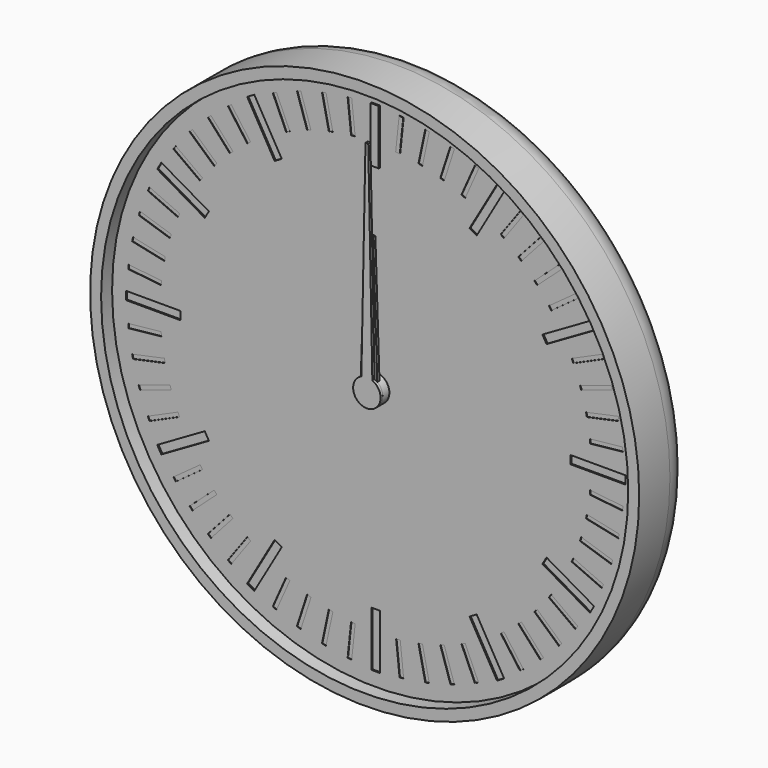
from build123d import *

# Parameters (mm, degrees)
F0_R      = 100
F1_DEPTH  = 24
F2_R      = 10
F3_T      = -4
F4_R      = 5
F4_R_2    = 3
F5_DEPTH  = 2
F6_DEPTH  = 19
F7_DEPTH  = 8
F9_DEPTH  = 4
F11_DEPTH = 4
F12_R     = 5
F12_R_2   = 3
F13_DEPTH = 2
F14_R     = 3
F15_DEPTH = 4
F17_DEPTH = 4
F18_R     = 3
F19_DEPTH = 2
F20_R     = 98
F20_R_2   = 5
F21_DEPTH = 1
F23_R     = 5
F23_R_2   = 3
F24_DEPTH = 2
F25_W     = 3
F25_H     = 20
F25_W_2   = 20
F25_H_2   = 3
F26_DEPTH = 0.5
F27_W     = 1.5
F27_H     = 12
F27_W_2   = 12
F27_H_2   = 1.5
F28_DEPTH = 0.2
F29_DEPTH = 1
F30_DEPTH = 0.4
F31_R     = 5
F31_R_2   = 3
F32_DEPTH = 5
F33_R     = 3
F34_DEPTH = 1
F36_DEPTH = 1


with BuildPart() as f1:
    # F0 (on Front) → F1 (new body)
    with BuildSketch(Plane.XZ):
        Circle(F0_R)
    extrude(amount=F1_DEPTH)

    # F2
    f2_edges = [f1.edges().sort_by_distance(p)[0] for p in [
        (-100, 0, 0),
    ]]
    fillet(f2_edges, radius=F2_R)

    # F3
    f3_openings = [f1.faces().sort_by_distance(p)[0] for p in [
        (0, -24, 0),
    ]]
    offset(amount=F3_T, openings=f3_openings)

    # F4 (on face) → F5 (join)
    with BuildSketch(Plane.XZ.offset(4)):
        Circle(F4_R)
        Circle(F4_R_2, mode=Mode.SUBTRACT)
        with Locations((40, 0)):
            Circle(F4_R)
        with Locations((40, 0)):
            Circle(F4_R_2, mode=Mode.SUBTRACT)
    extrude(amount=F5_DEPTH)


with BuildPart() as f6:
    # F6 (new): a face of the model
    f6_faces = [f1.part.faces().sort_by_distance(p)[0] for p in [
        (0, -4, 0),
    ]]
    extrude(f6_faces, amount=F6_DEPTH)

    # F8 (on face) → F9 (join)
    with BuildSketch(Plane.XZ.offset(6)):
        with BuildLine():
            ThreePointArc((9.2729637667, -1.3794085621), (9.3494561423, -0.6915886375), (9.375, 0))
            ThreePointArc((9.375, 0), (9.3494561423, 0.6915886375), (9.2729637667, 1.3794085621))
            ThreePointArc((9.2729637667, 1.3794085621), (8.9161548403, 2.8970343223), (8.3127812852, 4.3345463782))
            ThreePointArc((8.3127812852, 4.3345463782), (7.5845343223, 5.5104867402), (6.6911892658, 6.566476316))
            ThreePointArc((6.6911892658, 6.566476316), (5.5104867402, 7.5845343223), (4.1773988938, 8.3928519278))
            ThreePointArc((4.1773988938, 8.3928519278), (2.8970343223, 8.9161548403), (1.5536078905, 9.2453733036))
            ThreePointArc((1.5536078905, 9.2453733036), (0, 9.375), (-1.5536078905, 9.2453733036))
            ThreePointArc((-1.5536078905, 9.2453733036), (-2.8970343223, 8.9161548403), (-4.1773988938, 8.3928519278))
            ThreePointArc((-4.1773988938, 8.3928519278), (-5.5104867402, 7.5845343223), (-6.6911892658, 6.566476316))
            ThreePointArc((-6.6911892658, 6.566476316), (-7.5845343223, 5.5104867402), (-8.3127812852, 4.3345463782))
            ThreePointArc((-8.3127812852, 4.3345463782), (-8.9161548403, 2.8970343223), (-9.2729637667, 1.3794085621))
            ThreePointArc((-9.2729637667, 1.3794085621), (-9.375, 0), (-9.2729637667, -1.3794085621))
            ThreePointArc((-9.2729637667, -1.3794085621), (-8.9161548403, -2.8970343223), (-8.3127812852, -4.3345463782))
            ThreePointArc((-8.3127812852, -4.3345463782), (-7.5845343223, -5.5104867402), (-6.6911892658, -6.566476316))
            ThreePointArc((-6.6911892658, -6.566476316), (-5.5104867402, -7.5845343223), (-4.1773988938, -8.3928519278))
            ThreePointArc((-4.1773988938, -8.3928519278), (-2.8970343223, -8.9161548403), (-1.5536078905, -9.2453733036))
            ThreePointArc((-1.5536078905, -9.2453733036), (0, -9.375), (1.5536078905, -9.2453733036))
            ThreePointArc((1.5536078905, -9.2453733036), (2.8970343223, -8.9161548403), (4.1773988938, -8.3928519278))
            ThreePointArc((4.1773988938, -8.3928519278), (5.5104867402, -7.5845343223), (6.6911892658, -6.566476316))
            ThreePointArc((6.6911892658, -6.566476316), (7.5845343223, -5.5104867402), (8.3127812852, -4.3345463782))
            ThreePointArc((8.3127812852, -4.3345463782), (8.9161548403, -2.8970343223), (9.2729637667, -1.3794085621))
        make_face()
        with BuildLine():
            ThreePointArc((8.3127812852, 4.3345463782), (8.9161548403, 2.8970343223), (9.2729637667, 1.3794085621))
            Line((9.2729637667, 1.3794085621), (11.1823199426, 2.3946312492))
            Line((11.1823199426, 2.3946312492), (10.8182678729, 3.515068311))
            Line((10.8182678729, 3.515068311), (10.4542158031, 4.6355053728))
            Line((10.4542158031, 4.6355053728), (8.3127812852, 4.3345463782))
        make_face()
        with BuildLine():
            Line((11.1823199426, -2.3946312492), (9.2729637667, -1.3794085621))
            ThreePointArc((9.2729637667, -1.3794085621), (8.9161548403, -2.8970343223), (8.3127812852, -4.3345463782))
            Line((8.3127812852, -4.3345463782), (10.4542158031, -4.6355053728))
            Line((10.4542158031, -4.6355053728), (10.8182678729, -3.515068311))
            Line((10.8182678729, -3.515068311), (11.1823199426, -2.3946312492))
        make_face()
        with BuildLine():
            ThreePointArc((4.1773988938, 8.3928519278), (5.5104867402, 7.5845343223), (6.6911892658, 6.566476316))
            Line((6.6911892658, 6.566476316), (7.6391579371, 8.5101001246))
            Line((7.6391579371, 8.5101001246), (6.6860572448, 9.202568311))
            Line((6.6860572448, 9.202568311), (5.7329565525, 9.8950364974))
            Line((5.7329565525, 9.8950364974), (4.1773988938, 8.3928519278))
        make_face()
        with BuildLine():
            Line((7.6391579371, -8.5101001246), (6.6911892658, -6.566476316))
            ThreePointArc((6.6911892658, -6.566476316), (5.5104867402, -7.5845343223), (4.1773988938, -8.3928519278))
            Line((4.1773988938, -8.3928519278), (5.7329565525, -9.8950364974))
            Line((5.7329565525, -9.8950364974), (6.6860572448, -9.202568311))
            Line((6.6860572448, -9.202568311), (7.6391579371, -8.5101001246))
        make_face()
        with BuildLine():
            ThreePointArc((-1.5536078905, 9.2453733036), (0, 9.375), (1.5536078905, 9.2453733036))
            Line((1.5536078905, 9.2453733036), (1.1780972451, 11.375))
            Line((1.1780972451, 11.375), (0, 11.375))
            Line((0, 11.375), (-1.1780972451, 11.375))
            Line((-1.1780972451, 11.375), (-1.5536078905, 9.2453733036))
        make_face()
        with BuildLine():
            Line((1.1780972451, -11.375), (1.5536078905, -9.2453733036))
            ThreePointArc((1.5536078905, -9.2453733036), (0, -9.375), (-1.5536078905, -9.2453733036))
            Line((-1.5536078905, -9.2453733036), (-1.1780972451, -11.375))
            Line((-1.1780972451, -11.375), (0, -11.375))
            Line((0, -11.375), (1.1780972451, -11.375))
        make_face()
        with BuildLine():
            ThreePointArc((-6.6911892658, 6.566476316), (-5.5104867402, 7.5845343223), (-4.1773988938, 8.3928519278))
            Line((-4.1773988938, 8.3928519278), (-5.7329565525, 9.8950364974))
            Line((-5.7329565525, 9.8950364974), (-6.6860572448, 9.202568311))
            Line((-6.6860572448, 9.202568311), (-7.6391579371, 8.5101001246))
            Line((-7.6391579371, 8.5101001246), (-6.6911892658, 6.566476316))
        make_face()
        with BuildLine():
            Line((-5.7329565525, -9.8950364974), (-4.1773988938, -8.3928519278))
            ThreePointArc((-4.1773988938, -8.3928519278), (-5.5104867402, -7.5845343223), (-6.6911892658, -6.566476316))
            Line((-6.6911892658, -6.566476316), (-7.6391579371, -8.5101001246))
            Line((-7.6391579371, -8.5101001246), (-6.6860572448, -9.202568311))
            Line((-6.6860572448, -9.202568311), (-5.7329565525, -9.8950364974))
        make_face()
        with BuildLine():
            ThreePointArc((-9.2729637667, 1.3794085621), (-8.9161548403, 2.8970343223), (-8.3127812852, 4.3345463782))
            Line((-8.3127812852, 4.3345463782), (-10.4542158031, 4.6355053728))
            Line((-10.4542158031, 4.6355053728), (-10.8182678729, 3.515068311))
            Line((-10.8182678729, 3.515068311), (-11.1823199426, 2.3946312492))
            Line((-11.1823199426, 2.3946312492), (-9.2729637667, 1.3794085621))
        make_face()
        with BuildLine():
            Line((-10.4542158031, -4.6355053728), (-8.3127812852, -4.3345463782))
            ThreePointArc((-8.3127812852, -4.3345463782), (-8.9161548403, -2.8970343223), (-9.2729637667, -1.3794085621))
            Line((-9.2729637667, -1.3794085621), (-11.1823199426, -2.3946312492))
            Line((-11.1823199426, -2.3946312492), (-10.8182678729, -3.515068311))
            Line((-10.8182678729, -3.515068311), (-10.4542158031, -4.6355053728))
        make_face()
    extrude(amount=F9_DEPTH)

    # F35 (on face) → F36 (join)
    with BuildSketch(Plane.XZ.offset(23)):
        with BuildLine():
            ThreePointArc((-2, 4.582575695), (-2.7386127875, -4.1833001327), (5, 0))
            ThreePointArc((5, 0), (4.1833001327, 2.7386127875), (2, 4.582575695))
            ThreePointArc((2, 4.582575695), (0, 5), (-2, 4.582575695))
        make_face()
        with BuildLine():
            ThreePointArc((-2, 4.582575695), (0, 5), (2, 4.582575695))
            Line((2, 4.582575695), (0.5, 80))
            Line((0.5, 80), (0, 80))
            Line((0, 80), (-0.5, 80))
            Line((-0.5, 80), (-2, 4.582575695))
        make_face()
    extrude(amount=-F36_DEPTH)


with BuildPart() as f7:
    # F7 (new): a face of the model
    f7_faces = [f1.part.faces().sort_by_distance(p)[0] for p in [
        (40, -4, 0),
    ]]
    extrude(f7_faces, amount=F7_DEPTH)

    # F10 (on face) → F11 (join)
    with BuildSketch(Plane.XZ.offset(6)):
        with BuildLine():
            ThreePointArc((68.0829066802, -1.5381733945), (68.1144747006, -0.7693746225), (68.125, 0))
            ThreePointArc((68.125, 0), (68.1144747006, 0.7693746225), (68.0829066802, 1.5381733945))
            ThreePointArc((68.0829066802, 1.5381733945), (67.9709283072, 2.9398630294), (67.7890320221, 4.3342039956))
            ThreePointArc((67.7890320221, 4.3342039956), (67.5104012706, 5.8475163042), (67.1494235596, 7.3433252263))
            ThreePointArc((67.1494235596, 7.3433252263), (66.7484645208, 8.6911029668), (66.280643318, 10.0171558733))
            ThreePointArc((66.280643318, 10.0171558733), (65.6934659962, 11.4394680865), (65.0293803521, 12.8275385085))
            ThreePointArc((65.0293803521, 12.8275385085), (64.3569644814, 14.0625), (63.6236643925, 15.2623099717))
            ThreePointArc((63.6236643925, 15.2623099717), (62.7536029668, 16.5314602207), (61.815433119, 17.7511268046))
            ThreePointArc((61.815433119, 17.7511268046), (60.9009482166, 18.8192983038), (59.934217974, 19.8404278876))
            ThreePointArc((59.934217974, 19.8404278876), (58.8192983038, 20.9009482166), (57.6480467764, 21.8989056799))
            ThreePointArc((57.6480467764, 21.8989056799), (56.5314602207, 22.7536029668), (55.3735505752, 23.5514238999))
            ThreePointArc((55.3735505752, 23.5514238999), (54.0625, 24.3569644814), (52.709356105, 25.0895972944))
            ThreePointArc((52.709356105, 25.0895972944), (51.4394680865, 25.6934659962), (50.1409852457, 26.2331096755))
            ThreePointArc((50.1409852457, 26.2331096755), (48.6911029668, 26.7484645208), (47.2152055856, 27.1837531139))
            ThreePointArc((47.2152055856, 27.1837531139), (45.8475163042, 27.5104012706), (44.4652101991, 27.7682826779))
            ThreePointArc((44.4652101991, 27.7682826779), (42.9398630294, 27.9709283072), (41.4057159597, 28.0898484802))
            ThreePointArc((41.4057159597, 28.0898484802), (40, 28.125), (38.5942840403, 28.0898484802))
            ThreePointArc((38.5942840403, 28.0898484802), (37.0601369706, 27.9709283072), (35.5347898009, 27.7682826779))
            ThreePointArc((35.5347898009, 27.7682826779), (34.1524836958, 27.5104012706), (32.7847944144, 27.1837531139))
            ThreePointArc((32.7847944144, 27.1837531139), (31.3088970332, 26.7484645208), (29.8590147543, 26.2331096755))
            ThreePointArc((29.8590147543, 26.2331096755), (28.5605319135, 25.6934659962), (27.290643895, 25.0895972944))
            ThreePointArc((27.290643895, 25.0895972944), (25.9375, 24.3569644814), (24.6264494248, 23.5514238999))
            ThreePointArc((24.6264494248, 23.5514238999), (23.4685397793, 22.7536029668), (22.3519532236, 21.8989056799))
            ThreePointArc((22.3519532236, 21.8989056799), (21.1807016962, 20.9009482166), (20.065782026, 19.8404278876))
            ThreePointArc((20.065782026, 19.8404278876), (19.0990517834, 18.8192983038), (18.184566881, 17.7511268046))
            ThreePointArc((18.184566881, 17.7511268046), (17.2463970332, 16.5314602207), (16.3763356075, 15.2623099717))
            ThreePointArc((16.3763356075, 15.2623099717), (15.6430355186, 14.0625), (14.9706196479, 12.8275385085))
            ThreePointArc((14.9706196479, 12.8275385085), (14.3065340038, 11.4394680865), (13.719356682, 10.0171558733))
            ThreePointArc((13.719356682, 10.0171558733), (13.2515354792, 8.6911029668), (12.8505764404, 7.3433252263))
            ThreePointArc((12.8505764404, 7.3433252263), (12.4895987294, 5.8475163042), (12.2109679779, 4.3342039956))
            ThreePointArc((12.2109679779, 4.3342039956), (12.0290716928, 2.9398630294), (11.9170933198, 1.5381733945))
            ThreePointArc((11.9170933198, 1.5381733945), (11.875, 0), (11.9170933198, -1.5381733945))
            ThreePointArc((11.9170933198, -1.5381733945), (12.0290716928, -2.9398630294), (12.2109679779, -4.3342039956))
            ThreePointArc((12.2109679779, -4.3342039956), (12.4895987294, -5.8475163042), (12.8505764404, -7.3433252263))
            ThreePointArc((12.8505764404, -7.3433252263), (13.2515354792, -8.6911029668), (13.719356682, -10.0171558733))
            ThreePointArc((13.719356682, -10.0171558733), (14.3065340038, -11.4394680865), (14.9706196479, -12.8275385085))
            ThreePointArc((14.9706196479, -12.8275385085), (15.6430355186, -14.0625), (16.3763356075, -15.2623099717))
            ThreePointArc((16.3763356075, -15.2623099717), (17.2463970332, -16.5314602207), (18.184566881, -17.7511268046))
            ThreePointArc((18.184566881, -17.7511268046), (19.0990517834, -18.8192983038), (20.065782026, -19.8404278876))
            ThreePointArc((20.065782026, -19.8404278876), (21.1807016962, -20.9009482166), (22.3519532236, -21.8989056799))
            ThreePointArc((22.3519532236, -21.8989056799), (23.4685397793, -22.7536029668), (24.6264494248, -23.5514238999))
            ThreePointArc((24.6264494248, -23.5514238999), (25.9375, -24.3569644814), (27.290643895, -25.0895972944))
            ThreePointArc((27.290643895, -25.0895972944), (28.5605319135, -25.6934659962), (29.8590147543, -26.2331096755))
            ThreePointArc((29.8590147543, -26.2331096755), (31.3088970332, -26.7484645208), (32.7847944144, -27.1837531139))
            ThreePointArc((32.7847944144, -27.1837531139), (34.1524836958, -27.5104012706), (35.5347898009, -27.7682826779))
            ThreePointArc((35.5347898009, -27.7682826779), (37.0601369706, -27.9709283072), (38.5942840403, -28.0898484802))
            ThreePointArc((38.5942840403, -28.0898484802), (40, -28.125), (41.4057159597, -28.0898484802))
            ThreePointArc((41.4057159597, -28.0898484802), (42.9398630294, -27.9709283072), (44.4652101991, -27.7682826779))
            ThreePointArc((44.4652101991, -27.7682826779), (45.8475163042, -27.5104012706), (47.2152055856, -27.1837531139))
            ThreePointArc((47.2152055856, -27.1837531139), (48.6911029668, -26.7484645208), (50.1409852457, -26.2331096755))
            ThreePointArc((50.1409852457, -26.2331096755), (51.4394680865, -25.6934659962), (52.709356105, -25.0895972944))
            ThreePointArc((52.709356105, -25.0895972944), (54.0625, -24.3569644814), (55.3735505752, -23.5514238999))
            ThreePointArc((55.3735505752, -23.5514238999), (56.5314602207, -22.7536029668), (57.6480467764, -21.8989056799))
            ThreePointArc((57.6480467764, -21.8989056799), (58.8192983038, -20.9009482166), (59.934217974, -19.8404278876))
            ThreePointArc((59.934217974, -19.8404278876), (60.9009482166, -18.8192983038), (61.815433119, -17.7511268046))
            ThreePointArc((61.815433119, -17.7511268046), (62.7536029668, -16.5314602207), (63.6236643925, -15.2623099717))
            ThreePointArc((63.6236643925, -15.2623099717), (64.3569644814, -14.0625), (65.0293803521, -12.8275385085))
            ThreePointArc((65.0293803521, -12.8275385085), (65.6934659962, -11.4394680865), (66.280643318, -10.0171558733))
            ThreePointArc((66.280643318, -10.0171558733), (66.7484645208, -8.6911029668), (67.1494235596, -7.3433252263))
            ThreePointArc((67.1494235596, -7.3433252263), (67.5104012706, -5.8475163042), (67.7890320221, -4.3342039956))
            ThreePointArc((67.7890320221, -4.3342039956), (67.9709283072, -2.9398630294), (68.0829066802, -1.5381733945))
        make_face()
        with BuildLine():
            ThreePointArc((68.0829066802, 1.5381733945), (68.1144747006, 0.7693746225), (68.125, 0))
            ThreePointArc((68.125, 0), (68.1144747006, -0.7693746225), (68.0829066802, -1.5381733945))
            Line((68.0829066802, -1.5381733945), (70.125, -1.1780972451))
            Line((70.125, -1.1780972451), (70.125, 0))
            Line((70.125, 0), (70.125, 1.1780972451))
            Line((70.125, 1.1780972451), (68.0829066802, 1.5381733945))
        make_face()
        with BuildLine():
            ThreePointArc((67.1494235596, 7.3433252263), (67.5104012706, 5.8475163042), (67.7890320221, 4.3342039956))
            Line((67.7890320221, 4.3342039956), (69.7116366623, 5.1109866922))
            Line((69.7116366623, 5.1109866922), (69.4666964721, 6.2633396859))
            Line((69.4666964721, 6.2633396859), (69.2217562819, 7.4156926796))
            Line((69.2217562819, 7.4156926796), (67.1494235596, 7.3433252263))
        make_face()
        with BuildLine():
            Line((69.7116366623, -5.1109866922), (67.7890320221, -4.3342039956))
            ThreePointArc((67.7890320221, -4.3342039956), (67.5104012706, -5.8475163042), (67.1494235596, -7.3433252263))
            Line((67.1494235596, -7.3433252263), (69.2217562819, -7.4156926796))
            Line((69.2217562819, -7.4156926796), (69.4666964721, -6.2633396859))
            Line((69.4666964721, -6.2633396859), (69.7116366623, -5.1109866922))
        make_face()
        with BuildLine():
            ThreePointArc((65.0293803521, 12.8275385085), (65.6934659962, 11.4394680865), (66.280643318, 10.0171558733))
            Line((66.280643318, 10.0171558733), (67.9997322302, 11.1766959857))
            Line((67.9997322302, 11.1766959857), (67.5205569115, 12.2529413727))
            Line((67.5205569115, 12.2529413727), (67.0413815928, 13.3291867596))
            Line((67.0413815928, 13.3291867596), (65.0293803521, 12.8275385085))
        make_face()
        with BuildLine():
            Line((67.9997322302, -11.1766959857), (66.280643318, -10.0171558733))
            ThreePointArc((66.280643318, -10.0171558733), (65.6934659962, -11.4394680865), (65.0293803521, -12.8275385085))
            Line((65.0293803521, -12.8275385085), (67.0413815928, -13.3291867596))
            Line((67.0413815928, -13.3291867596), (67.5205569115, -12.2529413727))
            Line((67.5205569115, -12.2529413727), (67.9997322302, -11.1766959857))
        make_face()
        with BuildLine():
            ThreePointArc((61.815433119, 17.7511268046), (62.7536029668, 16.5314602207), (63.6236643925, 15.2623099717))
            Line((63.6236643925, 15.2623099717), (65.064105142, 16.753930033))
            Line((65.064105142, 16.753930033), (64.3716369555, 17.7070307253))
            Line((64.3716369555, 17.7070307253), (63.6791687691, 18.6601314176))
            Line((63.6791687691, 18.6601314176), (61.815433119, 17.7511268046))
        make_face()
        with BuildLine():
            Line((65.064105142, -16.753930033), (63.6236643925, -15.2623099717))
            ThreePointArc((63.6236643925, -15.2623099717), (62.7536029668, -16.5314602207), (61.815433119, -17.7511268046))
            Line((61.815433119, -17.7511268046), (63.6791687691, -18.6601314176))
            Line((63.6791687691, -18.6601314176), (64.3716369555, -17.7070307253))
            Line((64.3716369555, -17.7070307253), (65.064105142, -16.753930033))
        make_face()
        with BuildLine():
            ThreePointArc((57.6480467764, 21.8989056799), (58.8192983038, 20.9009482166), (59.934217974, 19.8404278876))
            Line((59.934217974, 19.8404278876), (61.0330563882, 21.5989369435))
            Line((61.0330563882, 21.5989369435), (60.1575595166, 22.3872378675))
            Line((60.1575595166, 22.3872378675), (59.282062645, 23.1755387915))
            Line((59.282062645, 23.1755387915), (57.6480467764, 21.8989056799))
        make_face()
        with BuildLine():
            Line((61.0330563882, -21.5989369435), (59.934217974, -19.8404278876))
            ThreePointArc((59.934217974, -19.8404278876), (58.8192983038, -20.9009482166), (57.6480467764, -21.8989056799))
            Line((57.6480467764, -21.8989056799), (59.282062645, -23.1755387915))
            Line((59.282062645, -23.1755387915), (60.1575595166, -22.3872378675))
            Line((60.1575595166, -22.3872378675), (61.0330563882, -21.5989369435))
        make_face()
        with BuildLine():
            ThreePointArc((52.709356105, 25.0895972944), (54.0625, 24.3569644814), (55.3735505752, 23.5514238999))
            Line((55.3735505752, 23.5514238999), (56.0827621424, 25.4999666665))
            Line((56.0827621424, 25.4999666665), (55.0625, 26.089015289))
            Line((55.0625, 26.089015289), (54.0422378576, 26.6780639116))
            Line((54.0422378576, 26.6780639116), (52.709356105, 25.0895972944))
        make_face()
        with BuildLine():
            Line((56.0827621424, -25.4999666665), (55.3735505752, -23.5514238999))
            ThreePointArc((55.3735505752, -23.5514238999), (54.0625, -24.3569644814), (52.709356105, -25.0895972944))
            Line((52.709356105, -25.0895972944), (54.0422378576, -26.6780639116))
            Line((54.0422378576, -26.6780639116), (55.0625, -26.089015289))
            Line((55.0625, -26.089015289), (56.0827621424, -25.4999666665))
        make_face()
        with BuildLine():
            ThreePointArc((47.2152055856, 27.1837531139), (48.6911029668, 26.7484645208), (50.1409852457, 26.2331096755))
            Line((50.1409852457, 26.2331096755), (50.4295740173, 28.2865254836))
            Line((50.4295740173, 28.2865254836), (49.3091369555, 28.6505775534))
            Line((49.3091369555, 28.6505775534), (48.1886998938, 29.0146296232))
            Line((48.1886998938, 29.0146296232), (47.2152055856, 27.1837531139))
        make_face()
        with BuildLine():
            Line((50.4295740173, -28.2865254836), (50.1409852457, -26.2331096755))
            ThreePointArc((50.1409852457, -26.2331096755), (48.6911029668, -26.7484645208), (47.2152055856, -27.1837531139))
            Line((47.2152055856, -27.1837531139), (48.1886998938, -29.0146296232))
            Line((48.1886998938, -29.0146296232), (49.3091369555, -28.6505775534))
            Line((49.3091369555, -28.6505775534), (50.4295740173, -28.2865254836))
        make_face()
        with BuildLine():
            ThreePointArc((41.4057159597, 28.0898484802), (42.9398630294, 27.9709283072), (44.4652101991, 27.7682826779))
            Line((44.4652101991, 27.7682826779), (44.3205634611, 29.8368274034))
            Line((44.3205634611, 29.8368274034), (43.1489199559, 29.959972098))
            Line((43.1489199559, 29.959972098), (41.9772764508, 30.0831167926))
            Line((41.9772764508, 30.0831167926), (41.4057159597, 28.0898484802))
        make_face()
        with BuildLine():
            Line((44.3205634611, -29.8368274034), (44.4652101991, -27.7682826779))
            ThreePointArc((44.4652101991, -27.7682826779), (42.9398630294, -27.9709283072), (41.4057159597, -28.0898484802))
            Line((41.4057159597, -28.0898484802), (41.9772764508, -30.0831167926))
            Line((41.9772764508, -30.0831167926), (43.1489199559, -29.959972098))
            Line((43.1489199559, -29.959972098), (44.3205634611, -29.8368274034))
        make_face()
        with BuildLine():
            ThreePointArc((35.5347898009, 27.7682826779), (37.0601369706, 27.9709283072), (38.5942840403, 28.0898484802))
            Line((38.5942840403, 28.0898484802), (38.0227235492, 30.0831167926))
            Line((38.0227235492, 30.0831167926), (36.8510800441, 29.959972098))
            Line((36.8510800441, 29.959972098), (35.6794365389, 29.8368274034))
            Line((35.6794365389, 29.8368274034), (35.5347898009, 27.7682826779))
        make_face()
        with BuildLine():
            Line((38.0227235492, -30.0831167926), (38.5942840403, -28.0898484802))
            ThreePointArc((38.5942840403, -28.0898484802), (37.0601369706, -27.9709283072), (35.5347898009, -27.7682826779))
            Line((35.5347898009, -27.7682826779), (35.6794365389, -29.8368274034))
            Line((35.6794365389, -29.8368274034), (36.8510800441, -29.959972098))
            Line((36.8510800441, -29.959972098), (38.0227235492, -30.0831167926))
        make_face()
        with BuildLine():
            ThreePointArc((29.8590147543, 26.2331096755), (31.3088970332, 26.7484645208), (32.7847944144, 27.1837531139))
            Line((32.7847944144, 27.1837531139), (31.8113001062, 29.0146296232))
            Line((31.8113001062, 29.0146296232), (30.6908630445, 28.6505775534))
            Line((30.6908630445, 28.6505775534), (29.5704259827, 28.2865254836))
            Line((29.5704259827, 28.2865254836), (29.8590147543, 26.2331096755))
        make_face()
        with BuildLine():
            Line((31.8113001062, -29.0146296232), (32.7847944144, -27.1837531139))
            ThreePointArc((32.7847944144, -27.1837531139), (31.3088970332, -26.7484645208), (29.8590147543, -26.2331096755))
            Line((29.8590147543, -26.2331096755), (29.5704259827, -28.2865254836))
            Line((29.5704259827, -28.2865254836), (30.6908630445, -28.6505775534))
            Line((30.6908630445, -28.6505775534), (31.8113001062, -29.0146296232))
        make_face()
        with BuildLine():
            ThreePointArc((24.6264494248, 23.5514238999), (25.9375, 24.3569644814), (27.290643895, 25.0895972944))
            Line((27.290643895, 25.0895972944), (25.9577621424, 26.6780639116))
            Line((25.9577621424, 26.6780639116), (24.9375, 26.089015289))
            Line((24.9375, 26.089015289), (23.9172378576, 25.4999666665))
            Line((23.9172378576, 25.4999666665), (24.6264494248, 23.5514238999))
        make_face()
        with BuildLine():
            Line((25.9577621424, -26.6780639116), (27.290643895, -25.0895972944))
            ThreePointArc((27.290643895, -25.0895972944), (25.9375, -24.3569644814), (24.6264494248, -23.5514238999))
            Line((24.6264494248, -23.5514238999), (23.9172378576, -25.4999666665))
            Line((23.9172378576, -25.4999666665), (24.9375, -26.089015289))
            Line((24.9375, -26.089015289), (25.9577621424, -26.6780639116))
        make_face()
        with BuildLine():
            ThreePointArc((20.065782026, 19.8404278876), (21.1807016962, 20.9009482166), (22.3519532236, 21.8989056799))
            Line((22.3519532236, 21.8989056799), (20.717937355, 23.1755387915))
            Line((20.717937355, 23.1755387915), (19.8424404834, 22.3872378675))
            Line((19.8424404834, 22.3872378675), (18.9669436118, 21.5989369435))
            Line((18.9669436118, 21.5989369435), (20.065782026, 19.8404278876))
        make_face()
        with BuildLine():
            Line((20.717937355, -23.1755387915), (22.3519532236, -21.8989056799))
            ThreePointArc((22.3519532236, -21.8989056799), (21.1807016962, -20.9009482166), (20.065782026, -19.8404278876))
            Line((20.065782026, -19.8404278876), (18.9669436118, -21.5989369435))
            Line((18.9669436118, -21.5989369435), (19.8424404834, -22.3872378675))
            Line((19.8424404834, -22.3872378675), (20.717937355, -23.1755387915))
        make_face()
        with BuildLine():
            ThreePointArc((16.3763356075, 15.2623099717), (17.2463970332, 16.5314602207), (18.184566881, 17.7511268046))
            Line((18.184566881, 17.7511268046), (16.3208312309, 18.6601314176))
            Line((16.3208312309, 18.6601314176), (15.6283630445, 17.7070307253))
            Line((15.6283630445, 17.7070307253), (14.935894858, 16.753930033))
            Line((14.935894858, 16.753930033), (16.3763356075, 15.2623099717))
        make_face()
        with BuildLine():
            Line((16.3208312309, -18.6601314176), (18.184566881, -17.7511268046))
            ThreePointArc((18.184566881, -17.7511268046), (17.2463970332, -16.5314602207), (16.3763356075, -15.2623099717))
            Line((16.3763356075, -15.2623099717), (14.935894858, -16.753930033))
            Line((14.935894858, -16.753930033), (15.6283630445, -17.7070307253))
            Line((15.6283630445, -17.7070307253), (16.3208312309, -18.6601314176))
        make_face()
        with BuildLine():
            ThreePointArc((13.719356682, 10.0171558733), (14.3065340038, 11.4394680865), (14.9706196479, 12.8275385085))
            Line((14.9706196479, 12.8275385085), (12.9586184072, 13.3291867596))
            Line((12.9586184072, 13.3291867596), (12.4794430885, 12.2529413727))
            Line((12.4794430885, 12.2529413727), (12.0002677698, 11.1766959857))
            Line((12.0002677698, 11.1766959857), (13.719356682, 10.0171558733))
        make_face()
        with BuildLine():
            Line((12.9586184072, -13.3291867596), (14.9706196479, -12.8275385085))
            ThreePointArc((14.9706196479, -12.8275385085), (14.3065340038, -11.4394680865), (13.719356682, -10.0171558733))
            Line((13.719356682, -10.0171558733), (12.0002677698, -11.1766959857))
            Line((12.0002677698, -11.1766959857), (12.4794430885, -12.2529413727))
            Line((12.4794430885, -12.2529413727), (12.9586184072, -13.3291867596))
        make_face()
        with BuildLine():
            ThreePointArc((12.2109679779, 4.3342039956), (12.4895987294, 5.8475163042), (12.8505764404, 7.3433252263))
            Line((12.8505764404, 7.3433252263), (10.7782437181, 7.4156926796))
            Line((10.7782437181, 7.4156926796), (10.5333035279, 6.2633396859))
            Line((10.5333035279, 6.2633396859), (10.2883633377, 5.1109866922))
            Line((10.2883633377, 5.1109866922), (12.2109679779, 4.3342039956))
        make_face()
        with BuildLine():
            Line((10.7782437181, -7.4156926796), (12.8505764404, -7.3433252263))
            ThreePointArc((12.8505764404, -7.3433252263), (12.4895987294, -5.8475163042), (12.2109679779, -4.3342039956))
            Line((12.2109679779, -4.3342039956), (10.2883633377, -5.1109866922))
            Line((10.2883633377, -5.1109866922), (10.5333035279, -6.2633396859))
            Line((10.5333035279, -6.2633396859), (10.7782437181, -7.4156926796))
        make_face()
        with BuildLine():
            ThreePointArc((11.9170933198, -1.5381733945), (11.875, 0), (11.9170933198, 1.5381733945))
            Line((11.9170933198, 1.5381733945), (9.875, 1.1780972451))
            Line((9.875, 1.1780972451), (9.875, 0))
            Line((9.875, 0), (9.875, -1.1780972451))
            Line((9.875, -1.1780972451), (11.9170933198, -1.5381733945))
        make_face()
    extrude(amount=F11_DEPTH)

    # F16 (on face) → F17 (join)
    with BuildSketch(Plane.XZ.offset(12)):
        with BuildLine():
            ThreePointArc((47.4288750323, -1.0304444454), (47.4821976298, -0.5164480894), (47.5, 0))
            ThreePointArc((47.5, 0), (47.4821976298, 0.5164480894), (47.4288750323, 1.0304444454))
            ThreePointArc((47.4288750323, 1.0304444454), (47.1329238722, 2.3176274578), (46.6157661985, 3.532936117))
            ThreePointArc((46.6157661985, 3.532936117), (46.0676274578, 4.4083893922), (45.4044061018, 5.2002302532))
            ThreePointArc((45.4044061018, 5.2002302532), (44.4083893922, 6.0676274578), (43.2756595386, 6.7468551628))
            ThreePointArc((43.2756595386, 6.7468551628), (42.3176274578, 7.1329238722), (41.3156377295, 7.3837048536))
            ThreePointArc((41.3156377295, 7.3837048536), (40, 7.5), (38.6843622705, 7.3837048536))
            ThreePointArc((38.6843622705, 7.3837048536), (37.6823725422, 7.1329238722), (36.7243404614, 6.7468551628))
            ThreePointArc((36.7243404614, 6.7468551628), (35.5916106078, 6.0676274578), (34.5955938982, 5.2002302532))
            ThreePointArc((34.5955938982, 5.2002302532), (33.9323725422, 4.4083893922), (33.3842338015, 3.532936117))
            ThreePointArc((33.3842338015, 3.532936117), (32.8670761278, 2.3176274578), (32.5711249677, 1.0304444454))
            ThreePointArc((32.5711249677, 1.0304444454), (32.5, 0), (32.5711249677, -1.0304444454))
            ThreePointArc((32.5711249677, -1.0304444454), (32.8670761278, -2.3176274578), (33.3842338015, -3.532936117))
            ThreePointArc((33.3842338015, -3.532936117), (33.9323725422, -4.4083893922), (34.5955938982, -5.2002302532))
            ThreePointArc((34.5955938982, -5.2002302532), (35.5916106078, -6.0676274578), (36.7243404614, -6.7468551628))
            ThreePointArc((36.7243404614, -6.7468551628), (37.6823725422, -7.1329238722), (38.6843622705, -7.3837048536))
            ThreePointArc((38.6843622705, -7.3837048536), (40, -7.5), (41.3156377295, -7.3837048536))
            ThreePointArc((41.3156377295, -7.3837048536), (42.3176274578, -7.1329238722), (43.2756595386, -6.7468551628))
            ThreePointArc((43.2756595386, -6.7468551628), (44.4083893922, -6.0676274578), (45.4044061018, -5.2002302532))
            ThreePointArc((45.4044061018, -5.2002302532), (46.0676274578, -4.4083893922), (46.6157661985, -3.532936117))
            ThreePointArc((46.6157661985, -3.532936117), (47.1329238722, -2.3176274578), (47.4288750323, -1.0304444454))
        make_face()
        with BuildLine():
            ThreePointArc((46.6157661985, 3.532936117), (47.1329238722, 2.3176274578), (47.4288750323, 1.0304444454))
            Line((47.4288750323, 1.0304444454), (49.3262785606, 2.0393117971))
            Line((49.3262785606, 2.0393117971), (49.0350369048, 2.9356614466))
            Line((49.0350369048, 2.9356614466), (48.743795249, 3.832011096))
            Line((48.743795249, 3.832011096), (46.6157661985, 3.532936117))
        make_face()
        with BuildLine():
            Line((49.3262785606, -2.0393117971), (47.4288750323, -1.0304444454))
            ThreePointArc((47.4288750323, -1.0304444454), (47.1329238722, -2.3176274578), (46.6157661985, -3.532936117))
            Line((46.6157661985, -3.532936117), (48.743795249, -3.832011096))
            Line((48.743795249, -3.832011096), (49.0350369048, -2.9356614466))
            Line((49.0350369048, -2.9356614466), (49.3262785606, -2.0393117971))
        make_face()
        with BuildLine():
            ThreePointArc((43.2756595386, 6.7468551628), (44.4083893922, 6.0676274578), (45.4044061018, 5.2002302532))
            Line((45.4044061018, 5.2002302532), (46.3464404506, 7.1316868974))
            Line((46.3464404506, 7.1316868974), (45.5839598968, 7.6856614466))
            Line((45.5839598968, 7.6856614466), (44.8214793429, 8.2396359957))
            Line((44.8214793429, 8.2396359957), (43.2756595386, 6.7468551628))
        make_face()
        with BuildLine():
            Line((46.3464404506, -7.1316868974), (45.4044061018, -5.2002302532))
            ThreePointArc((45.4044061018, -5.2002302532), (44.4083893922, -6.0676274578), (43.2756595386, -6.7468551628))
            Line((43.2756595386, -6.7468551628), (44.8214793429, -8.2396359957))
            Line((44.8214793429, -8.2396359957), (45.5839598968, -7.6856614466))
            Line((45.5839598968, -7.6856614466), (46.3464404506, -7.1316868974))
        make_face()
        with BuildLine():
            ThreePointArc((38.6843622705, 7.3837048536), (40, 7.5), (41.3156377295, 7.3837048536))
            Line((41.3156377295, 7.3837048536), (40.9424777961, 9.5))
            Line((40.9424777961, 9.5), (40, 9.5))
            Line((40, 9.5), (39.0575222039, 9.5))
            Line((39.0575222039, 9.5), (38.6843622705, 7.3837048536))
        make_face()
        with BuildLine():
            Line((40.9424777961, -9.5), (41.3156377295, -7.3837048536))
            ThreePointArc((41.3156377295, -7.3837048536), (40, -7.5), (38.6843622705, -7.3837048536))
            Line((38.6843622705, -7.3837048536), (39.0575222039, -9.5))
            Line((39.0575222039, -9.5), (40, -9.5))
            Line((40, -9.5), (40.9424777961, -9.5))
        make_face()
        with BuildLine():
            ThreePointArc((34.5955938982, 5.2002302532), (35.5916106078, 6.0676274578), (36.7243404614, 6.7468551628))
            Line((36.7243404614, 6.7468551628), (35.1785206571, 8.2396359957))
            Line((35.1785206571, 8.2396359957), (34.4160401032, 7.6856614466))
            Line((34.4160401032, 7.6856614466), (33.6535595494, 7.1316868974))
            Line((33.6535595494, 7.1316868974), (34.5955938982, 5.2002302532))
        make_face()
        with BuildLine():
            Line((35.1785206571, -8.2396359957), (36.7243404614, -6.7468551628))
            ThreePointArc((36.7243404614, -6.7468551628), (35.5916106078, -6.0676274578), (34.5955938982, -5.2002302532))
            Line((34.5955938982, -5.2002302532), (33.6535595494, -7.1316868974))
            Line((33.6535595494, -7.1316868974), (34.4160401032, -7.6856614466))
            Line((34.4160401032, -7.6856614466), (35.1785206571, -8.2396359957))
        make_face()
        with BuildLine():
            ThreePointArc((32.5711249677, 1.0304444454), (32.8670761278, 2.3176274578), (33.3842338015, 3.532936117))
            Line((33.3842338015, 3.532936117), (31.256204751, 3.832011096))
            Line((31.256204751, 3.832011096), (30.9649630952, 2.9356614466))
            Line((30.9649630952, 2.9356614466), (30.6737214394, 2.0393117971))
            Line((30.6737214394, 2.0393117971), (32.5711249677, 1.0304444454))
        make_face()
        with BuildLine():
            Line((31.256204751, -3.832011096), (33.3842338015, -3.532936117))
            ThreePointArc((33.3842338015, -3.532936117), (32.8670761278, -2.3176274578), (32.5711249677, -1.0304444454))
            Line((32.5711249677, -1.0304444454), (30.6737214394, -2.0393117971))
            Line((30.6737214394, -2.0393117971), (30.9649630952, -2.9356614466))
            Line((30.9649630952, -2.9356614466), (31.256204751, -3.832011096))
        make_face()
    extrude(amount=F17_DEPTH)

    # F18 (on face) → F19 (join)
    with BuildSketch(Plane.XZ.offset(16)):
        with Locations((40, 0)):
            Circle(F18_R)
    extrude(amount=F19_DEPTH)


with BuildPart() as f13:
    # F12 (on face) → F13 (new body)
    with BuildSketch(Plane.XZ.offset(10)):
        Circle(F12_R)
        Circle(F12_R_2, mode=Mode.SUBTRACT)
    extrude(amount=F13_DEPTH)

    # F14 (on face) → F15 (join)
    with BuildSketch(Plane.XZ.offset(12)):
        with BuildLine():
            ThreePointArc((29.9583421574, -1.580422468), (29.9895837311, -0.7904856977), (30, 0))
            ThreePointArc((30, 0), (29.9895837311, 0.7904856977), (29.9583421574, 1.580422468))
            ThreePointArc((29.9583421574, 1.580422468), (29.907520012, 2.3537728718), (29.8367377958, 3.1255523841))
            ThreePointArc((29.8367377958, 3.1255523841), (29.6306502179, 4.6930339512), (29.3422727092, 6.2474820737))
            ThreePointArc((29.3422727092, 6.2474820737), (29.1710976119, 7.0033609157), (28.9804539271, 7.7545657633))
            ThreePointArc((28.9804539271, 7.7545657633), (28.5316954889, 9.2705098312), (28.0036991253, 10.7607079366))
            ThreePointArc((28.0036991253, 10.7607079366), (27.7163859753, 11.480502971), (27.4105751022, 12.1926359975))
            ThreePointArc((27.4105751022, 12.1926359975), (26.7301957257, 13.6197149922), (25.9755815301, 15.0089694574))
            ThreePointArc((25.9755815301, 15.0089694574), (25.5792049306, 15.6749569415), (25.1657569477, 16.3304830684))
            ThreePointArc((25.1657569477, 16.3304830684), (24.2705098312, 17.6335575688), (23.3078589096, 18.8876603382))
            ThreePointArc((23.3078589096, 18.8876603382), (22.812178968, 19.4834414499), (22.3012743369, 20.0662194484))
            ThreePointArc((22.3012743369, 20.0662194484), (21.2132034356, 21.2132034356), (20.0662194484, 22.3012743369))
            ThreePointArc((20.0662194484, 22.3012743369), (19.4834414499, 22.812178968), (18.8876603382, 23.3078589096))
            ThreePointArc((18.8876603382, 23.3078589096), (17.6335575688, 24.2705098312), (16.3304830684, 25.1657569477))
            ThreePointArc((16.3304830684, 25.1657569477), (15.6749569415, 25.5792049306), (15.0089694574, 25.9755815301))
            ThreePointArc((15.0089694574, 25.9755815301), (13.6197149922, 26.7301957257), (12.1926359975, 27.4105751022))
            ThreePointArc((12.1926359975, 27.4105751022), (11.480502971, 27.7163859753), (10.7607079366, 28.0036991253))
            ThreePointArc((10.7607079366, 28.0036991253), (9.2705098312, 28.5316954889), (7.7545657633, 28.9804539271))
            ThreePointArc((7.7545657633, 28.9804539271), (7.0033609157, 29.1710976119), (6.2474820737, 29.3422727092))
            ThreePointArc((6.2474820737, 29.3422727092), (4.6930339512, 29.6306502179), (3.1255523841, 29.8367377958))
            ThreePointArc((3.1255523841, 29.8367377958), (2.3537728718, 29.907520012), (1.580422468, 29.9583421574))
            ThreePointArc((1.580422468, 29.9583421574), (0, 30), (-1.580422468, 29.9583421574))
            ThreePointArc((-1.580422468, 29.9583421574), (-2.3537728718, 29.907520012), (-3.1255523841, 29.8367377958))
            ThreePointArc((-3.1255523841, 29.8367377958), (-4.6930339512, 29.6306502179), (-6.2474820737, 29.3422727092))
            ThreePointArc((-6.2474820737, 29.3422727092), (-7.0033609157, 29.1710976119), (-7.7545657633, 28.9804539271))
            ThreePointArc((-7.7545657633, 28.9804539271), (-9.2705098312, 28.5316954889), (-10.7607079366, 28.0036991253))
            ThreePointArc((-10.7607079366, 28.0036991253), (-11.480502971, 27.7163859753), (-12.1926359975, 27.4105751022))
            ThreePointArc((-12.1926359975, 27.4105751022), (-13.6197149922, 26.7301957257), (-15.0089694574, 25.9755815301))
            ThreePointArc((-15.0089694574, 25.9755815301), (-15.6749569415, 25.5792049306), (-16.3304830684, 25.1657569477))
            ThreePointArc((-16.3304830684, 25.1657569477), (-17.6335575688, 24.2705098312), (-18.8876603382, 23.3078589096))
            ThreePointArc((-18.8876603382, 23.3078589096), (-19.4834414499, 22.812178968), (-20.0662194484, 22.3012743369))
            ThreePointArc((-20.0662194484, 22.3012743369), (-21.2132034356, 21.2132034356), (-22.3012743369, 20.0662194484))
            ThreePointArc((-22.3012743369, 20.0662194484), (-22.812178968, 19.4834414499), (-23.3078589096, 18.8876603382))
            ThreePointArc((-23.3078589096, 18.8876603382), (-24.2705098312, 17.6335575688), (-25.1657569477, 16.3304830684))
            ThreePointArc((-25.1657569477, 16.3304830684), (-25.5792049306, 15.6749569415), (-25.9755815301, 15.0089694574))
            ThreePointArc((-25.9755815301, 15.0089694574), (-26.7301957257, 13.6197149922), (-27.4105751022, 12.1926359975))
            ThreePointArc((-27.4105751022, 12.1926359975), (-27.7163859753, 11.480502971), (-28.0036991253, 10.7607079366))
            ThreePointArc((-28.0036991253, 10.7607079366), (-28.5316954889, 9.2705098312), (-28.9804539271, 7.7545657633))
            ThreePointArc((-28.9804539271, 7.7545657633), (-29.1710976119, 7.0033609157), (-29.3422727092, 6.2474820737))
            ThreePointArc((-29.3422727092, 6.2474820737), (-29.6306502179, 4.6930339512), (-29.8367377958, 3.1255523841))
            ThreePointArc((-29.8367377958, 3.1255523841), (-29.907520012, 2.3537728718), (-29.9583421574, 1.580422468))
            ThreePointArc((-29.9583421574, 1.580422468), (-30, 0), (-29.9583421574, -1.580422468))
            ThreePointArc((-29.9583421574, -1.580422468), (-29.907520012, -2.3537728718), (-29.8367377958, -3.1255523841))
            ThreePointArc((-29.8367377958, -3.1255523841), (-29.6306502179, -4.6930339512), (-29.3422727092, -6.2474820737))
            ThreePointArc((-29.3422727092, -6.2474820737), (-29.1710976119, -7.0033609157), (-28.9804539271, -7.7545657633))
            ThreePointArc((-28.9804539271, -7.7545657633), (-28.5316954889, -9.2705098312), (-28.0036991253, -10.7607079366))
            ThreePointArc((-28.0036991253, -10.7607079366), (-27.7163859753, -11.480502971), (-27.4105751022, -12.1926359975))
            ThreePointArc((-27.4105751022, -12.1926359975), (-26.7301957257, -13.6197149922), (-25.9755815301, -15.0089694574))
            ThreePointArc((-25.9755815301, -15.0089694574), (-25.5792049306, -15.6749569415), (-25.1657569477, -16.3304830684))
            ThreePointArc((-25.1657569477, -16.3304830684), (-24.2705098312, -17.6335575688), (-23.3078589096, -18.8876603382))
            ThreePointArc((-23.3078589096, -18.8876603382), (-22.812178968, -19.4834414499), (-22.3012743369, -20.0662194484))
            ThreePointArc((-22.3012743369, -20.0662194484), (-21.2132034356, -21.2132034356), (-20.0662194484, -22.3012743369))
            ThreePointArc((-20.0662194484, -22.3012743369), (-19.4834414499, -22.812178968), (-18.8876603382, -23.3078589096))
            ThreePointArc((-18.8876603382, -23.3078589096), (-17.6335575688, -24.2705098312), (-16.3304830684, -25.1657569477))
            ThreePointArc((-16.3304830684, -25.1657569477), (-15.6749569415, -25.5792049306), (-15.0089694574, -25.9755815301))
            ThreePointArc((-15.0089694574, -25.9755815301), (-13.6197149922, -26.7301957257), (-12.1926359975, -27.4105751022))
            ThreePointArc((-12.1926359975, -27.4105751022), (-11.480502971, -27.7163859753), (-10.7607079366, -28.0036991253))
            ThreePointArc((-10.7607079366, -28.0036991253), (-9.2705098312, -28.5316954889), (-7.7545657633, -28.9804539271))
            ThreePointArc((-7.7545657633, -28.9804539271), (-7.0033609157, -29.1710976119), (-6.2474820737, -29.3422727092))
            ThreePointArc((-6.2474820737, -29.3422727092), (-4.6930339512, -29.6306502179), (-3.1255523841, -29.8367377958))
            ThreePointArc((-3.1255523841, -29.8367377958), (-2.3537728718, -29.907520012), (-1.580422468, -29.9583421574))
            ThreePointArc((-1.580422468, -29.9583421574), (0, -30), (1.580422468, -29.9583421574))
            ThreePointArc((1.580422468, -29.9583421574), (2.3537728718, -29.907520012), (3.1255523841, -29.8367377958))
            ThreePointArc((3.1255523841, -29.8367377958), (4.6930339512, -29.6306502179), (6.2474820737, -29.3422727092))
            ThreePointArc((6.2474820737, -29.3422727092), (7.0033609157, -29.1710976119), (7.7545657633, -28.9804539271))
            ThreePointArc((7.7545657633, -28.9804539271), (9.2705098312, -28.5316954889), (10.7607079366, -28.0036991253))
            ThreePointArc((10.7607079366, -28.0036991253), (11.480502971, -27.7163859753), (12.1926359975, -27.4105751022))
            ThreePointArc((12.1926359975, -27.4105751022), (13.6197149922, -26.7301957257), (15.0089694574, -25.9755815301))
            ThreePointArc((15.0089694574, -25.9755815301), (15.6749569415, -25.5792049306), (16.3304830684, -25.1657569477))
            ThreePointArc((16.3304830684, -25.1657569477), (17.6335575688, -24.2705098312), (18.8876603382, -23.3078589096))
            ThreePointArc((18.8876603382, -23.3078589096), (19.4834414499, -22.812178968), (20.0662194484, -22.3012743369))
            ThreePointArc((20.0662194484, -22.3012743369), (21.2132034356, -21.2132034356), (22.3012743369, -20.0662194484))
            ThreePointArc((22.3012743369, -20.0662194484), (22.812178968, -19.4834414499), (23.3078589096, -18.8876603382))
            ThreePointArc((23.3078589096, -18.8876603382), (24.2705098312, -17.6335575688), (25.1657569477, -16.3304830684))
            ThreePointArc((25.1657569477, -16.3304830684), (25.5792049306, -15.6749569415), (25.9755815301, -15.0089694574))
            ThreePointArc((25.9755815301, -15.0089694574), (26.7301957257, -13.6197149922), (27.4105751022, -12.1926359975))
            ThreePointArc((27.4105751022, -12.1926359975), (27.7163859753, -11.480502971), (28.0036991253, -10.7607079366))
            ThreePointArc((28.0036991253, -10.7607079366), (28.5316954889, -9.2705098312), (28.9804539271, -7.7545657633))
            ThreePointArc((28.9804539271, -7.7545657633), (29.1710976119, -7.0033609157), (29.3422727092, -6.2474820737))
            ThreePointArc((29.3422727092, -6.2474820737), (29.6306502179, -4.6930339512), (29.8367377958, -3.1255523841))
            ThreePointArc((29.8367377958, -3.1255523841), (29.907520012, -2.3537728718), (29.9583421574, -1.580422468))
        make_face()
        Circle(F14_R, mode=Mode.SUBTRACT)
        with BuildLine():
            ThreePointArc((29.9583421574, 1.580422468), (29.9895837311, 0.7904856977), (30, 0))
            ThreePointArc((30, 0), (29.9895837311, -0.7904856977), (29.9583421574, -1.580422468))
            Line((29.9583421574, -1.580422468), (32, -0.9424777961))
            Line((32, -0.9424777961), (32, 0))
            Line((32, 0), (32, 0.9424777961))
            Line((32, 0.9424777961), (29.9583421574, 1.580422468))
        make_face()
        with BuildLine():
            ThreePointArc((29.3422727092, 6.2474820737), (29.6306502179, 4.6930339512), (29.8367377958, 3.1255523841))
            Line((29.8367377958, 3.1255523841), (31.7534629089, 4.0750285508))
            Line((31.7534629089, 4.0750285508), (31.606026899, 5.0059028813))
            Line((31.606026899, 5.0059028813), (31.4585908892, 5.9367772117))
            Line((31.4585908892, 5.9367772117), (29.3422727092, 6.2474820737))
        make_face()
        with BuildLine():
            Line((31.7534629089, -4.0750285508), (29.8367377958, -3.1255523841))
            ThreePointArc((29.8367377958, -3.1255523841), (29.6306502179, -4.6930339512), (29.3422727092, -6.2474820737))
            Line((29.3422727092, -6.2474820737), (31.4585908892, -5.9367772117))
            Line((31.4585908892, -5.9367772117), (31.606026899, -5.0059028813))
            Line((31.606026899, -5.0059028813), (31.7534629089, -4.0750285508))
        make_face()
        with BuildLine():
            ThreePointArc((28.0036991253, 10.7607079366), (28.5316954889, 9.2705098312), (28.9804539271, 7.7545657633))
            Line((28.9804539271, 7.7545657633), (30.7250501773, 8.9921941706))
            Line((30.7250501773, 8.9921941706), (30.4338085214, 9.88854382))
            Line((30.4338085214, 9.88854382), (30.1425668656, 10.7848934694))
            Line((30.1425668656, 10.7848934694), (28.0036991253, 10.7607079366))
        make_face()
        with BuildLine():
            Line((30.7250501773, -8.9921941706), (28.9804539271, -7.7545657633))
            ThreePointArc((28.9804539271, -7.7545657633), (28.5316954889, -9.2705098312), (28.0036991253, -10.7607079366))
            Line((28.0036991253, -10.7607079366), (30.1425668656, -10.7848934694))
            Line((30.1425668656, -10.7848934694), (30.4338085214, -9.88854382))
            Line((30.4338085214, -9.88854382), (30.7250501773, -8.9921941706))
        make_face()
        with BuildLine():
            ThreePointArc((25.9755815301, 15.0089694574), (26.7301957257, 13.6197149922), (27.4105751022, 12.1926359975))
            Line((27.4105751022, 12.1926359975), (28.9400847397, 13.6879421265))
            Line((28.9400847397, 13.6879421265), (28.512208774, 14.5276959917))
            Line((28.512208774, 14.5276959917), (28.0843328084, 15.3674498569))
            Line((28.0843328084, 15.3674498569), (25.9755815301, 15.0089694574))
        make_face()
        with BuildLine():
            Line((28.9400847397, -13.6879421265), (27.4105751022, -12.1926359975))
            ThreePointArc((27.4105751022, -12.1926359975), (26.7301957257, -13.6197149922), (25.9755815301, -15.0089694574))
            Line((25.9755815301, -15.0089694574), (28.0843328084, -15.3674498569))
            Line((28.0843328084, -15.3674498569), (28.512208774, -14.5276959917))
            Line((28.512208774, -14.5276959917), (28.9400847397, -13.6879421265))
        make_face()
        with BuildLine():
            ThreePointArc((23.3078589096, 18.8876603382), (24.2705098312, 17.6335575688), (25.1657569477, 16.3304830684))
            Line((25.1657569477, 16.3304830684), (26.4425183691, 18.0466475195))
            Line((26.4425183691, 18.0466475195), (25.88854382, 18.8091280734))
            Line((25.88854382, 18.8091280734), (25.3345692709, 19.5716086272))
            Line((25.3345692709, 19.5716086272), (23.3078589096, 18.8876603382))
        make_face()
        with BuildLine():
            Line((26.4425183691, -18.0466475195), (25.1657569477, -16.3304830684))
            ThreePointArc((25.1657569477, -16.3304830684), (24.2705098312, -17.6335575688), (23.3078589096, -18.8876603382))
            Line((23.3078589096, -18.8876603382), (25.3345692709, -19.5716086272))
            Line((25.3345692709, -19.5716086272), (25.88854382, -18.8091280734))
            Line((25.88854382, -18.8091280734), (26.4425183691, -18.0466475195))
        make_face()
        with BuildLine():
            ThreePointArc((20.0662194484, 22.3012743369), (21.2132034356, 21.2132034356), (22.3012743369, 20.0662194484))
            Line((22.3012743369, 20.0662194484), (23.2938494387, 21.9609845572))
            Line((23.2938494387, 21.9609845572), (22.627416998, 22.627416998))
            Line((22.627416998, 22.627416998), (21.9609845572, 23.2938494387))
            Line((21.9609845572, 23.2938494387), (20.0662194484, 22.3012743369))
        make_face()
        with BuildLine():
            Line((23.2938494387, -21.9609845572), (22.3012743369, -20.0662194484))
            ThreePointArc((22.3012743369, -20.0662194484), (21.2132034356, -21.2132034356), (20.0662194484, -22.3012743369))
            Line((20.0662194484, -22.3012743369), (21.9609845572, -23.2938494387))
            Line((21.9609845572, -23.2938494387), (22.627416998, -22.627416998))
            Line((22.627416998, -22.627416998), (23.2938494387, -21.9609845572))
        make_face()
        with BuildLine():
            ThreePointArc((16.3304830684, 25.1657569477), (17.6335575688, 24.2705098312), (18.8876603382, 23.3078589096))
            Line((18.8876603382, 23.3078589096), (19.5716086272, 25.3345692709))
            Line((19.5716086272, 25.3345692709), (18.8091280734, 25.88854382))
            Line((18.8091280734, 25.88854382), (18.0466475195, 26.4425183691))
            Line((18.0466475195, 26.4425183691), (16.3304830684, 25.1657569477))
        make_face()
        with BuildLine():
            Line((19.5716086272, -25.3345692709), (18.8876603382, -23.3078589096))
            ThreePointArc((18.8876603382, -23.3078589096), (17.6335575688, -24.2705098312), (16.3304830684, -25.1657569477))
            Line((16.3304830684, -25.1657569477), (18.0466475195, -26.4425183691))
            Line((18.0466475195, -26.4425183691), (18.8091280734, -25.88854382))
            Line((18.8091280734, -25.88854382), (19.5716086272, -25.3345692709))
        make_face()
        with BuildLine():
            ThreePointArc((12.1926359975, 27.4105751022), (13.6197149922, 26.7301957257), (15.0089694574, 25.9755815301))
            Line((15.0089694574, 25.9755815301), (15.3674498569, 28.0843328084))
            Line((15.3674498569, 28.0843328084), (14.5276959917, 28.512208774))
            Line((14.5276959917, 28.512208774), (13.6879421265, 28.9400847397))
            Line((13.6879421265, 28.9400847397), (12.1926359975, 27.4105751022))
        make_face()
        with BuildLine():
            Line((15.3674498569, -28.0843328084), (15.0089694574, -25.9755815301))
            ThreePointArc((15.0089694574, -25.9755815301), (13.6197149922, -26.7301957257), (12.1926359975, -27.4105751022))
            Line((12.1926359975, -27.4105751022), (13.6879421265, -28.9400847397))
            Line((13.6879421265, -28.9400847397), (14.5276959917, -28.512208774))
            Line((14.5276959917, -28.512208774), (15.3674498569, -28.0843328084))
        make_face()
        with BuildLine():
            ThreePointArc((7.7545657633, 28.9804539271), (9.2705098312, 28.5316954889), (10.7607079366, 28.0036991253))
            Line((10.7607079366, 28.0036991253), (10.7848934694, 30.1425668656))
            Line((10.7848934694, 30.1425668656), (9.88854382, 30.4338085214))
            Line((9.88854382, 30.4338085214), (8.9921941706, 30.7250501773))
            Line((8.9921941706, 30.7250501773), (7.7545657633, 28.9804539271))
        make_face()
        with BuildLine():
            Line((10.7848934694, -30.1425668656), (10.7607079366, -28.0036991253))
            ThreePointArc((10.7607079366, -28.0036991253), (9.2705098312, -28.5316954889), (7.7545657633, -28.9804539271))
            Line((7.7545657633, -28.9804539271), (8.9921941706, -30.7250501773))
            Line((8.9921941706, -30.7250501773), (9.88854382, -30.4338085214))
            Line((9.88854382, -30.4338085214), (10.7848934694, -30.1425668656))
        make_face()
        with BuildLine():
            ThreePointArc((3.1255523841, 29.8367377958), (4.6930339512, 29.6306502179), (6.2474820737, 29.3422727092))
            Line((6.2474820737, 29.3422727092), (5.9367772117, 31.4585908892))
            Line((5.9367772117, 31.4585908892), (5.0059028813, 31.606026899))
            Line((5.0059028813, 31.606026899), (4.0750285508, 31.7534629089))
            Line((4.0750285508, 31.7534629089), (3.1255523841, 29.8367377958))
        make_face()
        with BuildLine():
            Line((5.9367772117, -31.4585908892), (6.2474820737, -29.3422727092))
            ThreePointArc((6.2474820737, -29.3422727092), (4.6930339512, -29.6306502179), (3.1255523841, -29.8367377958))
            Line((3.1255523841, -29.8367377958), (4.0750285508, -31.7534629089))
            Line((4.0750285508, -31.7534629089), (5.0059028813, -31.606026899))
            Line((5.0059028813, -31.606026899), (5.9367772117, -31.4585908892))
        make_face()
        with BuildLine():
            ThreePointArc((-1.580422468, 29.9583421574), (0, 30), (1.580422468, 29.9583421574))
            Line((1.580422468, 29.9583421574), (0.9424777961, 32))
            Line((0.9424777961, 32), (0, 32))
            Line((0, 32), (-0.9424777961, 32))
            Line((-0.9424777961, 32), (-1.580422468, 29.9583421574))
        make_face()
        with BuildLine():
            Line((0.9424777961, -32), (1.580422468, -29.9583421574))
            ThreePointArc((1.580422468, -29.9583421574), (0, -30), (-1.580422468, -29.9583421574))
            Line((-1.580422468, -29.9583421574), (-0.9424777961, -32))
            Line((-0.9424777961, -32), (0, -32))
            Line((0, -32), (0.9424777961, -32))
        make_face()
        with BuildLine():
            ThreePointArc((-6.2474820737, 29.3422727092), (-4.6930339512, 29.6306502179), (-3.1255523841, 29.8367377958))
            Line((-3.1255523841, 29.8367377958), (-4.0750285508, 31.7534629089))
            Line((-4.0750285508, 31.7534629089), (-5.0059028813, 31.606026899))
            Line((-5.0059028813, 31.606026899), (-5.9367772117, 31.4585908892))
            Line((-5.9367772117, 31.4585908892), (-6.2474820737, 29.3422727092))
        make_face()
        with BuildLine():
            Line((-4.0750285508, -31.7534629089), (-3.1255523841, -29.8367377958))
            ThreePointArc((-3.1255523841, -29.8367377958), (-4.6930339512, -29.6306502179), (-6.2474820737, -29.3422727092))
            Line((-6.2474820737, -29.3422727092), (-5.9367772117, -31.4585908892))
            Line((-5.9367772117, -31.4585908892), (-5.0059028813, -31.606026899))
            Line((-5.0059028813, -31.606026899), (-4.0750285508, -31.7534629089))
        make_face()
        with BuildLine():
            ThreePointArc((-10.7607079366, 28.0036991253), (-9.2705098312, 28.5316954889), (-7.7545657633, 28.9804539271))
            Line((-7.7545657633, 28.9804539271), (-8.9921941706, 30.7250501773))
            Line((-8.9921941706, 30.7250501773), (-9.88854382, 30.4338085214))
            Line((-9.88854382, 30.4338085214), (-10.7848934694, 30.1425668656))
            Line((-10.7848934694, 30.1425668656), (-10.7607079366, 28.0036991253))
        make_face()
        with BuildLine():
            Line((-8.9921941706, -30.7250501773), (-7.7545657633, -28.9804539271))
            ThreePointArc((-7.7545657633, -28.9804539271), (-9.2705098312, -28.5316954889), (-10.7607079366, -28.0036991253))
            Line((-10.7607079366, -28.0036991253), (-10.7848934694, -30.1425668656))
            Line((-10.7848934694, -30.1425668656), (-9.88854382, -30.4338085214))
            Line((-9.88854382, -30.4338085214), (-8.9921941706, -30.7250501773))
        make_face()
        with BuildLine():
            ThreePointArc((-15.0089694574, 25.9755815301), (-13.6197149922, 26.7301957257), (-12.1926359975, 27.4105751022))
            Line((-12.1926359975, 27.4105751022), (-13.6879421265, 28.9400847397))
            Line((-13.6879421265, 28.9400847397), (-14.5276959917, 28.512208774))
            Line((-14.5276959917, 28.512208774), (-15.3674498569, 28.0843328084))
            Line((-15.3674498569, 28.0843328084), (-15.0089694574, 25.9755815301))
        make_face()
        with BuildLine():
            Line((-13.6879421265, -28.9400847397), (-12.1926359975, -27.4105751022))
            ThreePointArc((-12.1926359975, -27.4105751022), (-13.6197149922, -26.7301957257), (-15.0089694574, -25.9755815301))
            Line((-15.0089694574, -25.9755815301), (-15.3674498569, -28.0843328084))
            Line((-15.3674498569, -28.0843328084), (-14.5276959917, -28.512208774))
            Line((-14.5276959917, -28.512208774), (-13.6879421265, -28.9400847397))
        make_face()
        with BuildLine():
            ThreePointArc((-18.8876603382, 23.3078589096), (-17.6335575688, 24.2705098312), (-16.3304830684, 25.1657569477))
            Line((-16.3304830684, 25.1657569477), (-18.0466475195, 26.4425183691))
            Line((-18.0466475195, 26.4425183691), (-18.8091280734, 25.88854382))
            Line((-18.8091280734, 25.88854382), (-19.5716086272, 25.3345692709))
            Line((-19.5716086272, 25.3345692709), (-18.8876603382, 23.3078589096))
        make_face()
        with BuildLine():
            Line((-18.0466475195, -26.4425183691), (-16.3304830684, -25.1657569477))
            ThreePointArc((-16.3304830684, -25.1657569477), (-17.6335575688, -24.2705098312), (-18.8876603382, -23.3078589096))
            Line((-18.8876603382, -23.3078589096), (-19.5716086272, -25.3345692709))
            Line((-19.5716086272, -25.3345692709), (-18.8091280734, -25.88854382))
            Line((-18.8091280734, -25.88854382), (-18.0466475195, -26.4425183691))
        make_face()
        with BuildLine():
            ThreePointArc((-22.3012743369, 20.0662194484), (-21.2132034356, 21.2132034356), (-20.0662194484, 22.3012743369))
            Line((-20.0662194484, 22.3012743369), (-21.9609845572, 23.2938494387))
            Line((-21.9609845572, 23.2938494387), (-22.627416998, 22.627416998))
            Line((-22.627416998, 22.627416998), (-23.2938494387, 21.9609845572))
            Line((-23.2938494387, 21.9609845572), (-22.3012743369, 20.0662194484))
        make_face()
        with BuildLine():
            Line((-21.9609845572, -23.2938494387), (-20.0662194484, -22.3012743369))
            ThreePointArc((-20.0662194484, -22.3012743369), (-21.2132034356, -21.2132034356), (-22.3012743369, -20.0662194484))
            Line((-22.3012743369, -20.0662194484), (-23.2938494387, -21.9609845572))
            Line((-23.2938494387, -21.9609845572), (-22.627416998, -22.627416998))
            Line((-22.627416998, -22.627416998), (-21.9609845572, -23.2938494387))
        make_face()
        with BuildLine():
            ThreePointArc((-25.1657569477, 16.3304830684), (-24.2705098312, 17.6335575688), (-23.3078589096, 18.8876603382))
            Line((-23.3078589096, 18.8876603382), (-25.3345692709, 19.5716086272))
            Line((-25.3345692709, 19.5716086272), (-25.88854382, 18.8091280734))
            Line((-25.88854382, 18.8091280734), (-26.4425183691, 18.0466475195))
            Line((-26.4425183691, 18.0466475195), (-25.1657569477, 16.3304830684))
        make_face()
        with BuildLine():
            Line((-25.3345692709, -19.5716086272), (-23.3078589096, -18.8876603382))
            ThreePointArc((-23.3078589096, -18.8876603382), (-24.2705098312, -17.6335575688), (-25.1657569477, -16.3304830684))
            Line((-25.1657569477, -16.3304830684), (-26.4425183691, -18.0466475195))
            Line((-26.4425183691, -18.0466475195), (-25.88854382, -18.8091280734))
            Line((-25.88854382, -18.8091280734), (-25.3345692709, -19.5716086272))
        make_face()
        with BuildLine():
            ThreePointArc((-27.4105751022, 12.1926359975), (-26.7301957257, 13.6197149922), (-25.9755815301, 15.0089694574))
            Line((-25.9755815301, 15.0089694574), (-28.0843328084, 15.3674498569))
            Line((-28.0843328084, 15.3674498569), (-28.512208774, 14.5276959917))
            Line((-28.512208774, 14.5276959917), (-28.9400847397, 13.6879421265))
            Line((-28.9400847397, 13.6879421265), (-27.4105751022, 12.1926359975))
        make_face()
        with BuildLine():
            Line((-28.0843328084, -15.3674498569), (-25.9755815301, -15.0089694574))
            ThreePointArc((-25.9755815301, -15.0089694574), (-26.7301957257, -13.6197149922), (-27.4105751022, -12.1926359975))
            Line((-27.4105751022, -12.1926359975), (-28.9400847397, -13.6879421265))
            Line((-28.9400847397, -13.6879421265), (-28.512208774, -14.5276959917))
            Line((-28.512208774, -14.5276959917), (-28.0843328084, -15.3674498569))
        make_face()
        with BuildLine():
            ThreePointArc((-28.9804539271, 7.7545657633), (-28.5316954889, 9.2705098312), (-28.0036991253, 10.7607079366))
            Line((-28.0036991253, 10.7607079366), (-30.1425668656, 10.7848934694))
            Line((-30.1425668656, 10.7848934694), (-30.4338085214, 9.88854382))
            Line((-30.4338085214, 9.88854382), (-30.7250501773, 8.9921941706))
            Line((-30.7250501773, 8.9921941706), (-28.9804539271, 7.7545657633))
        make_face()
        with BuildLine():
            Line((-30.1425668656, -10.7848934694), (-28.0036991253, -10.7607079366))
            ThreePointArc((-28.0036991253, -10.7607079366), (-28.5316954889, -9.2705098312), (-28.9804539271, -7.7545657633))
            Line((-28.9804539271, -7.7545657633), (-30.7250501773, -8.9921941706))
            Line((-30.7250501773, -8.9921941706), (-30.4338085214, -9.88854382))
            Line((-30.4338085214, -9.88854382), (-30.1425668656, -10.7848934694))
        make_face()
        with BuildLine():
            ThreePointArc((-29.8367377958, 3.1255523841), (-29.6306502179, 4.6930339512), (-29.3422727092, 6.2474820737))
            Line((-29.3422727092, 6.2474820737), (-31.4585908892, 5.9367772117))
            Line((-31.4585908892, 5.9367772117), (-31.606026899, 5.0059028813))
            Line((-31.606026899, 5.0059028813), (-31.7534629089, 4.0750285508))
            Line((-31.7534629089, 4.0750285508), (-29.8367377958, 3.1255523841))
        make_face()
        with BuildLine():
            Line((-31.4585908892, -5.9367772117), (-29.3422727092, -6.2474820737))
            ThreePointArc((-29.3422727092, -6.2474820737), (-29.6306502179, -4.6930339512), (-29.8367377958, -3.1255523841))
            Line((-29.8367377958, -3.1255523841), (-31.7534629089, -4.0750285508))
            Line((-31.7534629089, -4.0750285508), (-31.606026899, -5.0059028813))
            Line((-31.606026899, -5.0059028813), (-31.4585908892, -5.9367772117))
        make_face()
        with BuildLine():
            ThreePointArc((-29.9583421574, -1.580422468), (-30, 0), (-29.9583421574, 1.580422468))
            Line((-29.9583421574, 1.580422468), (-32, 0.9424777961))
            Line((-32, 0.9424777961), (-32, 0))
            Line((-32, 0), (-32, -0.9424777961))
            Line((-32, -0.9424777961), (-29.9583421574, -1.580422468))
        make_face()
    extrude(amount=F15_DEPTH)

    # F31 (on face) → F32 (join)
    with BuildSketch(Plane.XZ.offset(16)):
        Circle(F31_R)
        Circle(F31_R_2, mode=Mode.SUBTRACT)
    extrude(amount=F32_DEPTH)

    # F33 (on face) → F34 (join)
    with BuildSketch(Plane.XZ.offset(21)):
        with BuildLine():
            ThreePointArc((-3, 4), (-2.2360679775, -4.472135955), (5, 0))
            ThreePointArc((5, 0), (4.472135955, 2.2360679775), (3, 4))
            ThreePointArc((3, 4), (0, 5), (-3, 4))
        make_face()
        Circle(F33_R, mode=Mode.SUBTRACT)
        with BuildLine():
            ThreePointArc((-3, 4), (0, 5), (3, 4))
            Line((3, 4), (1.5, 50))
            Line((1.5, 50), (0, 50))
            Line((0, 50), (-1.5, 50))
            Line((-1.5, 50), (-3, 4))
        make_face()
    extrude(amount=F34_DEPTH)


with BuildPart() as f21:
    # F20 (on face) → F21 (new body)
    with BuildSketch(Plane.XZ.offset(18)):
        Circle(F20_R)
        Circle(F20_R_2, mode=Mode.SUBTRACT)
    extrude(amount=F21_DEPTH)


with BuildPart() as f1_1:
    add(f1.part)

    # F22: cut F21
    add(f21.part, mode=Mode.SUBTRACT)


with BuildPart() as f21_1:
    add(f21.part)

    # F23 (on face) → F24 (join, through all)
    with BuildSketch(Plane(origin=(0, -18, 0), x_dir=(-1, 0, 0), z_dir=(0, 1, 0))):
        with Locations((-40, 0)):
            Circle(F23_R)
        with Locations((-40, 0)):
            Circle(F23_R_2, mode=Mode.SUBTRACT)
    extrude(amount=F24_DEPTH)

    # F25 (on face) → F26 (cut)
    with BuildSketch(Plane.XZ.offset(19)):
        with Locations((0, 81)):
            Rectangle(F25_W, F25_H)
        Polygon((-46.7990381057, 78.0583117444), (-36.7990381057, 60.7378036687), (-34.2009618943, 62.2378036687), (-44.2009618943, 79.5583117444), align=None)
        Polygon((-79.5583117444, 44.2009618943), (-62.2378036687, 34.2009618943), (-60.7378036687, 36.7990381057), (-78.0583117444, 46.7990381057), align=None)
        with Locations((-81, 0)):
            Rectangle(F25_W_2, F25_H_2)
        Polygon((-78.0583117444, -46.7990381057), (-60.7378036687, -36.7990381057), (-62.2378036687, -34.2009618943), (-79.5583117444, -44.2009618943), align=None)
        Polygon((-44.2009618943, -79.5583117444), (-34.2009618943, -62.2378036687), (-36.7990381057, -60.7378036687), (-46.7990381057, -78.0583117444), align=None)
        with Locations((0, -81)):
            Rectangle(F25_W, F25_H)
        Polygon((46.7990381057, -78.0583117444), (36.7990381057, -60.7378036687), (34.2009618943, -62.2378036687), (44.2009618943, -79.5583117444), align=None)
        Polygon((79.5583117444, -44.2009618943), (62.2378036687, -34.2009618943), (60.7378036687, -36.7990381057), (78.0583117444, -46.7990381057), align=None)
        with Locations((81, 0)):
            Rectangle(F25_W_2, F25_H_2)
        Polygon((78.0583117444, 46.7990381057), (60.7378036687, 36.7990381057), (62.2378036687, 34.2009618943), (79.5583117444, 44.2009618943), align=None)
        Polygon((44.2009618943, 79.5583117444), (34.2009618943, 62.2378036687), (36.7990381057, 60.7378036687), (46.7990381057, 78.0583117444), align=None)
    extrude(amount=-F26_DEPTH, mode=Mode.SUBTRACT)

    # F27 (on face) → F28 (cut)
    with BuildSketch(Plane.XZ.offset(19)):
        with Locations((0, 84.5)):
            Rectangle(F27_W, F27_H)
        Polygon((-10.2057173472, 89.9258351834), (-8.951375788, 77.991572439), (-7.459592945, 78.1483651339), (-8.7139345042, 90.0826278783), align=None)
        Polygon((-19.5496187196, 88.3664240983), (-17.0546784297, 76.6286528895), (-15.5874570286, 76.9405204257), (-18.0823973185, 88.6782916345), align=None)
        Polygon((-28.6793303782, 85.8388519789), (-24.9711264457, 74.4261737834), (-23.5445416712, 74.889699275), (-27.2527456037, 86.3023774705), align=None)
        Polygon((-37.4948252916, 82.3708114343), (-32.6139855747, 71.4082659426), (-31.2436673882, 72.0183709073), (-36.1245071051, 82.980916399), align=None)
        Polygon((-45.8995190528, 78.0002990425), (-39.8995190528, 67.6079941971), (-38.6004809472, 68.3579941971), (-44.6004809472, 78.7502990425), align=None)
        Polygon((-53.8013280783, 72.7751990517), (-46.7479050507, 63.0669951192), (-45.5343795592, 63.9486729977), (-52.5878025867, 73.6568769302), align=None)
        Polygon((-61.1136784946, 66.7527587509), (-53.0841112183, 57.8350208452), (-51.9693939801, 58.8387167547), (-59.9989612564, 67.7564546605), align=None)
        Polygon((-67.7564546605, 59.9989612564), (-58.8387167547, 51.9693939801), (-57.8350208452, 53.0841112183), (-66.7527587509, 61.1136784946), align=None)
        Polygon((-73.6568769302, 52.5878025867), (-63.9486729977, 45.5343795592), (-63.0669951192, 46.7479050507), (-72.7751990517, 53.8013280783), align=None)
        Polygon((-78.7502990425, 44.6004809472), (-68.3579941971, 38.6004809472), (-67.6079941971, 39.8995190528), (-78.0002990425, 45.8995190528), align=None)
        Polygon((-82.980916399, 36.1245071051), (-72.0183709073, 31.2436673882), (-71.4082659426, 32.6139855747), (-82.3708114343, 37.4948252916), align=None)
        Polygon((-86.3023774705, 27.2527456037), (-74.889699275, 23.5445416712), (-74.4261737834, 24.9711264457), (-85.8388519789, 28.6793303782), align=None)
        Polygon((-88.6782916345, 18.0823973185), (-76.9405204257, 15.5874570286), (-76.6286528895, 17.0546784297), (-88.3664240983, 19.5496187196), align=None)
        Polygon((-90.0826278783, 8.7139345042), (-78.1483651339, 7.459592945), (-77.991572439, 8.951375788), (-89.9258351834, 10.2057173472), align=None)
        with Locations((-84.5, 0)):
            Rectangle(F27_W_2, F27_H_2)
        Polygon((-89.9258351834, -10.2057173472), (-77.991572439, -8.951375788), (-78.1483651339, -7.459592945), (-90.0826278783, -8.7139345042), align=None)
        Polygon((-88.3664240983, -19.5496187196), (-76.6286528895, -17.0546784297), (-76.9405204257, -15.5874570286), (-88.6782916345, -18.0823973185), align=None)
        Polygon((-85.8388519789, -28.6793303782), (-74.4261737834, -24.9711264457), (-74.889699275, -23.5445416712), (-86.3023774705, -27.2527456037), align=None)
        Polygon((-82.3708114343, -37.4948252916), (-71.4082659426, -32.6139855747), (-72.0183709073, -31.2436673882), (-82.980916399, -36.1245071051), align=None)
        Polygon((-78.0002990425, -45.8995190528), (-67.6079941971, -39.8995190528), (-68.3579941971, -38.6004809472), (-78.7502990425, -44.6004809472), align=None)
        Polygon((-72.7751990517, -53.8013280783), (-63.0669951192, -46.7479050507), (-63.9486729977, -45.5343795592), (-73.6568769302, -52.5878025867), align=None)
        Polygon((-66.7527587509, -61.1136784946), (-57.8350208452, -53.0841112183), (-58.8387167547, -51.9693939801), (-67.7564546605, -59.9989612564), align=None)
        Polygon((-59.9989612564, -67.7564546605), (-51.9693939801, -58.8387167547), (-53.0841112183, -57.8350208452), (-61.1136784946, -66.7527587509), align=None)
        Polygon((-52.5878025867, -73.6568769302), (-45.5343795592, -63.9486729977), (-46.7479050507, -63.0669951192), (-53.8013280783, -72.7751990517), align=None)
        Polygon((-44.6004809472, -78.7502990425), (-38.6004809472, -68.3579941971), (-39.8995190528, -67.6079941971), (-45.8995190528, -78.0002990425), align=None)
        Polygon((-36.1245071051, -82.980916399), (-31.2436673882, -72.0183709073), (-32.6139855747, -71.4082659426), (-37.4948252916, -82.3708114343), align=None)
        Polygon((-27.2527456037, -86.3023774705), (-23.5445416712, -74.889699275), (-24.9711264457, -74.4261737834), (-28.6793303782, -85.8388519789), align=None)
        Polygon((-18.0823973185, -88.6782916345), (-15.5874570286, -76.9405204257), (-17.0546784297, -76.6286528895), (-19.5496187196, -88.3664240983), align=None)
        Polygon((-8.7139345042, -90.0826278783), (-7.459592945, -78.1483651339), (-8.951375788, -77.991572439), (-10.2057173472, -89.9258351834), align=None)
        with Locations((0, -84.5)):
            Rectangle(F27_W, F27_H)
        Polygon((10.2057173472, -89.9258351834), (8.951375788, -77.991572439), (7.459592945, -78.1483651339), (8.7139345042, -90.0826278783), align=None)
        Polygon((19.5496187196, -88.3664240983), (17.0546784297, -76.6286528895), (15.5874570286, -76.9405204257), (18.0823973185, -88.6782916345), align=None)
        Polygon((28.6793303782, -85.8388519789), (24.9711264457, -74.4261737834), (23.5445416712, -74.889699275), (27.2527456037, -86.3023774705), align=None)
        Polygon((37.4948252916, -82.3708114343), (32.6139855747, -71.4082659426), (31.2436673882, -72.0183709073), (36.1245071051, -82.980916399), align=None)
        Polygon((45.8995190528, -78.0002990425), (39.8995190528, -67.6079941971), (38.6004809472, -68.3579941971), (44.6004809472, -78.7502990425), align=None)
        Polygon((53.8013280783, -72.7751990517), (46.7479050507, -63.0669951192), (45.5343795592, -63.9486729977), (52.5878025867, -73.6568769302), align=None)
        Polygon((61.1136784946, -66.7527587509), (53.0841112183, -57.8350208452), (51.9693939801, -58.8387167547), (59.9989612564, -67.7564546605), align=None)
        Polygon((67.7564546605, -59.9989612564), (58.8387167547, -51.9693939801), (57.8350208452, -53.0841112183), (66.7527587509, -61.1136784946), align=None)
        Polygon((73.6568769302, -52.5878025867), (63.9486729977, -45.5343795592), (63.0669951192, -46.7479050507), (72.7751990517, -53.8013280783), align=None)
        Polygon((78.7502990425, -44.6004809472), (68.3579941971, -38.6004809472), (67.6079941971, -39.8995190528), (78.0002990425, -45.8995190528), align=None)
        Polygon((82.980916399, -36.1245071051), (72.0183709073, -31.2436673882), (71.4082659426, -32.6139855747), (82.3708114343, -37.4948252916), align=None)
        Polygon((86.3023774705, -27.2527456037), (74.889699275, -23.5445416712), (74.4261737834, -24.9711264457), (85.8388519789, -28.6793303782), align=None)
        Polygon((88.6782916345, -18.0823973185), (76.9405204257, -15.5874570286), (76.6286528895, -17.0546784297), (88.3664240983, -19.5496187196), align=None)
        Polygon((90.0826278783, -8.7139345042), (78.1483651339, -7.459592945), (77.991572439, -8.951375788), (89.9258351834, -10.2057173472), align=None)
        with Locations((84.5, 0)):
            Rectangle(F27_W_2, F27_H_2)
        Polygon((89.9258351834, 10.2057173472), (77.991572439, 8.951375788), (78.1483651339, 7.459592945), (90.0826278783, 8.7139345042), align=None)
        Polygon((88.3664240983, 19.5496187196), (76.6286528895, 17.0546784297), (76.9405204257, 15.5874570286), (88.6782916345, 18.0823973185), align=None)
        Polygon((85.8388519789, 28.6793303782), (74.4261737834, 24.9711264457), (74.889699275, 23.5445416712), (86.3023774705, 27.2527456037), align=None)
        Polygon((82.3708114343, 37.4948252916), (71.4082659426, 32.6139855747), (72.0183709073, 31.2436673882), (82.980916399, 36.1245071051), align=None)
        Polygon((78.0002990425, 45.8995190528), (67.6079941971, 39.8995190528), (68.3579941971, 38.6004809472), (78.7502990425, 44.6004809472), align=None)
        Polygon((72.7751990517, 53.8013280783), (63.0669951192, 46.7479050507), (63.9486729977, 45.5343795592), (73.6568769302, 52.5878025867), align=None)
        Polygon((66.7527587509, 61.1136784946), (57.8350208452, 53.0841112183), (58.8387167547, 51.9693939801), (67.7564546605, 59.9989612564), align=None)
        Polygon((59.9989612564, 67.7564546605), (51.9693939801, 58.8387167547), (53.0841112183, 57.8350208452), (61.1136784946, 66.7527587509), align=None)
        Polygon((52.5878025867, 73.6568769302), (45.5343795592, 63.9486729977), (46.7479050507, 63.0669951192), (53.8013280783, 72.7751990517), align=None)
        Polygon((44.6004809472, 78.7502990425), (38.6004809472, 68.3579941971), (39.8995190528, 67.6079941971), (45.8995190528, 78.0002990425), align=None)
        Polygon((36.1245071051, 82.980916399), (31.2436673882, 72.0183709073), (32.6139855747, 71.4082659426), (37.4948252916, 82.3708114343), align=None)
        Polygon((27.2527456037, 86.3023774705), (23.5445416712, 74.889699275), (24.9711264457, 74.4261737834), (28.6793303782, 85.8388519789), align=None)
        Polygon((18.0823973185, 88.6782916345), (15.5874570286, 76.9405204257), (17.0546784297, 76.6286528895), (19.5496187196, 88.3664240983), align=None)
        Polygon((8.7139345042, 90.0826278783), (7.459592945, 78.1483651339), (8.951375788, 77.991572439), (10.2057173472, 89.9258351834), align=None)
    extrude(amount=-F28_DEPTH, mode=Mode.SUBTRACT)


with BuildPart() as f29:
    # F29 (new): a face of the model
    f29_faces = [f21_1.part.faces().sort_by_distance(p)[0] for p in [
        (0, -18.5, 81),
    ]]
    extrude(f29_faces, amount=F29_DEPTH)


with BuildPart() as f30:
    # F30 (new): a face of the model
    f30_faces = [f21_1.part.faces().sort_by_distance(p)[0] for p in [
        (8.8326551461, -18.8, 84.0371001586),
    ]]
    extrude(f30_faces, amount=F30_DEPTH)


solid = Compound([f6.part, f7.part, f13.part, f1_1.part, f21_1.part, f29.part, f30.part])
